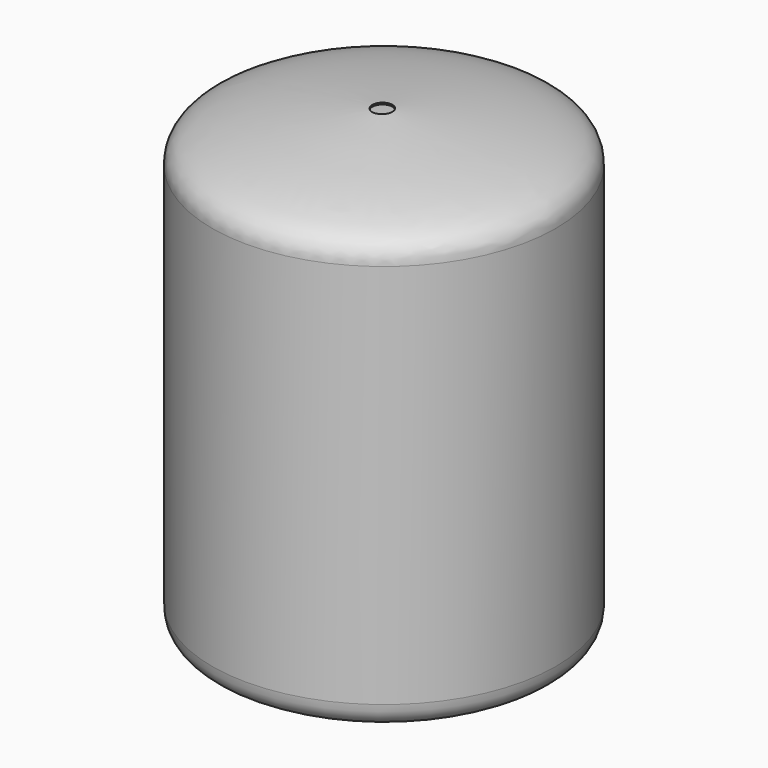
from build123d import *

# Parameters (mm, degrees)
F2_W = 1.4728322858
F2_H = 61.4517312497


# Not quite as in the source:
# - the dataset's text gives a spline's control points without its knots; the knots are read off the source's solid


with BuildPart() as f1:
    # F0 (on Front) → F1 (revolve)
    with BuildSketch(Plane.XZ):
        with BuildLine():
            Line((-24.8476303218, -23.6559781424), (-24.8476303218, 33.2400218576))
            add(Edge.make_bspline(
                [(-24.8476303218, 33.2400218576), (-24.8392485082, 35.0878313184), (-21.9392536265, 37.9085215783), (-9.2245090879, 39.6275790934), (0, 40.3551720083)],
                knots=[0, 0, 0, 0, 0.307284137, 1, 1, 1, 1], degree=3))
            Line((0, 40.3551720083), (-0.0199724864, 40.6083855541))
            add(Edge.make_bspline(
                [(-25.1016277087, 33.2411740104), (-25.099847883, 33.6335448075), (-25.0203220233, 34.3450092517), (-24.6535972704, 35.2288301982), (-24.0412005583, 35.9395252885), (-23.2103986691, 36.5092249364), (-22.1699081303, 36.9960600829), (-20.910119069, 37.4527536189), (-19.445095335, 37.8812292864), (-17.241866473, 38.4171752718), (-14.0636821492, 39.0228870029), (-9.7185440354, 39.6512229907), (-4.9916574994, 40.183899894), (-1.6861555728, 40.4769636002), (-0.0199724864, 40.6083855541)],
                knots=[0, 0, 0, 0, 0.0625, 0.125, 0.1874999999, 0.2499999999, 0.3124999999, 0.3749999999, 0.4374999999, 0.4999999998, 0.6249999998, 0.7499999997, 0.8749999997, 0.9999999997, 0.9999999997, 0.9999999997, 0.9999999997], degree=3))
            Line((-25.1016277087, 33.2411740104), (-25.1016303218, 33.2400218576))
            Line((-25.1016303218, 33.2400218576), (-25.1016303218, -23.6559781424))
            Line((-25.1016303218, -23.6559781424), (-25.1016277087, -23.6571302952))
            add(Edge.make_bspline(
                [(-25.1016277087, -23.6571302952), (-25.099847883, -24.0495010923), (-25.0203220233, -24.7609655365), (-24.6535972704, -25.644786483), (-24.0412005583, -26.3554815733), (-23.2103986691, -26.9251812212), (-22.1699081303, -27.4120163677), (-20.910119069, -27.8687099037), (-19.445095335, -28.2971855712), (-17.241866473, -28.8331315566), (-14.0636821492, -29.4388432877), (-9.7185440354, -30.0671792755), (-4.9916574994, -30.5998561788), (-1.6861555728, -30.892919885), (-0.0199724864, -31.0243418389)],
                knots=[0, 0, 0, 0, 0.0625, 0.125, 0.1874999999, 0.2499999999, 0.3124999999, 0.3749999999, 0.4374999999, 0.4999999998, 0.6249999998, 0.7499999997, 0.8749999997, 0.9999999997, 0.9999999997, 0.9999999997, 0.9999999997], degree=3))
            Line((-0.0199724864, -31.0243418389), (0, -30.7711282931))
            add(Edge.make_bspline(
                [(-24.8476303218, -23.6559781424), (-24.8392485082, -25.5037876032), (-21.9392536265, -28.3244778631), (-9.2245090879, -30.0435353782), (0, -30.7711282931)],
                knots=[0, 0, 0, 0, 0.307284137, 1, 1, 1, 1], degree=3))
        make_face()
    revolve(axis=Axis((0.254, 0, 5.0864014775), (0, 0, -1)))

    # F2 (on Front) → F3 (revolve, cut)
    with BuildSketch(Plane.XZ):
        with Locations((0.7364161429, 16.4334746078)):
            Rectangle(F2_W, F2_H)
    revolve(axis=Axis((0, 0, 16.4334746078), (0, 0, -1)), mode=Mode.SUBTRACT)


solid = f1.part
